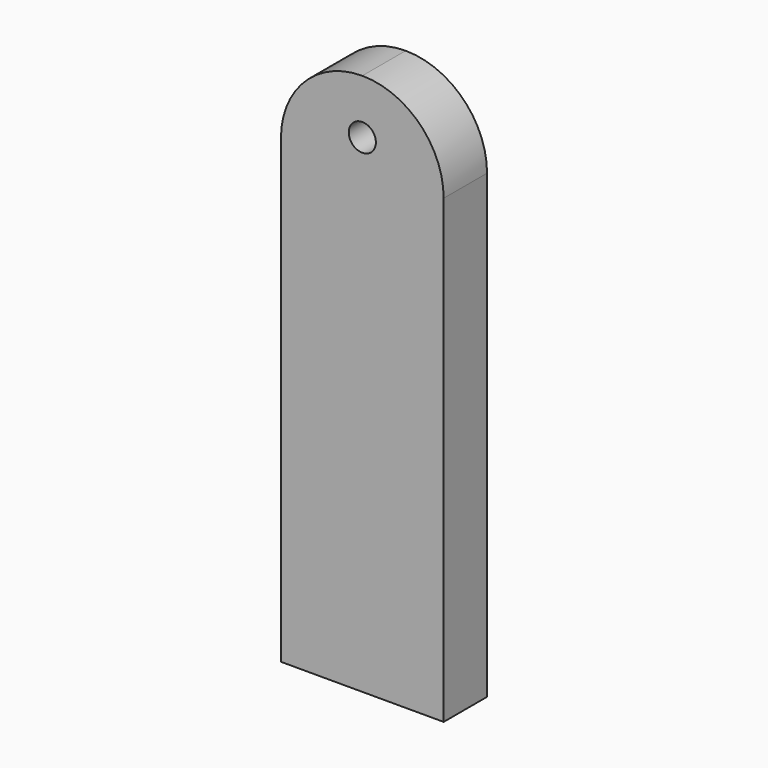
from build123d import *

# Parameters (mm, degrees)
F0_W     = 76.2
F0_H     = 254
F0_R     = 6.35
F1_DEPTH = 25.4
F2_R     = 38.09999


# Not quite as in the source:
# - a fillet or chamfer is up to 0.001 mm smaller than in the source, because OpenCascade refuses the exact size


with BuildPart() as f1:
    # F0 (on Front) → F1 (new body)
    with BuildSketch(Plane.XZ):
        with Locations((-38.1, 127)):
            Rectangle(F0_W, F0_H)
        with Locations((-38.1, 228.6)):
            Circle(F0_R, mode=Mode.SUBTRACT)
    extrude(amount=F1_DEPTH)

    # F2 (radius 38.1 in the source; OpenCascade refuses exactly that, so slightly less here)
    f2_edges = [f1.edges().sort_by_distance(p)[0] for p in [
        (-76.2, -12.7, 254),
        (0, -12.7, 254),
    ]]
    fillet(f2_edges, radius=F2_R)


solid = f1.part
